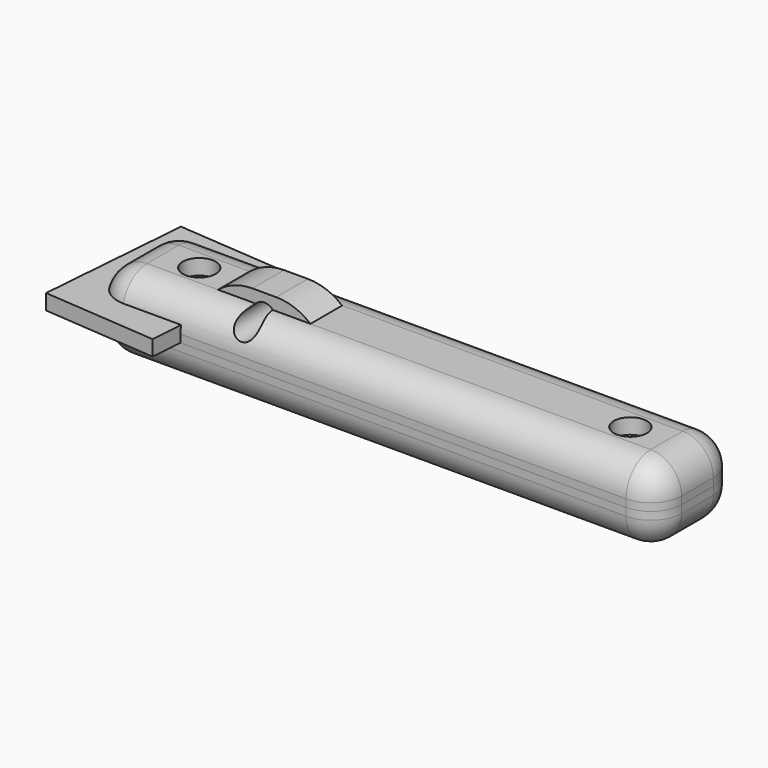
from build123d import *

# Parameters (mm, degrees)
F1_DEPTH    = 2.54
F2_R        = 1.905
F3_DEPTH    = 6.35
F4_DEPTH    = 6.35
F5_R        = 5.08
F6_R        = 5.08
F7_W        = 15.24
F7_H        = 6.5325613847
F8_DEPTH    = 2.032
F9_T1_DEPTH = 34.8168043479
F11_D       = 3.81
F11_DEPTH   = 5.0913193076
F12_D       = 3.81
F14_D       = 5.461
F14_DEPTH   = 2.54
F14_TIP     = 1.6406499203
F15_R       = 1.905
F16_DEPTH   = 4.064


# Not quite as in the source:
# - a fillet or chamfer that OpenCascade refuses, or shapes differently, is made with other operations: its cross-section is extruded or revolved along the edge and cut away or added
# - a feature of the source that left no trace in its solid (it failed there, or was rolled back) is left out


with BuildPart() as f1:
    # F0 (on Top) → F1 (new body)
    with BuildSketch(Plane.XY):
        Polygon((-30.4073522295, 11.7323991549), (-49.1452058091, 13.2097140262), (-50.143391533, 0.5490021481), (-51.1415772568, -12.11170973), (-32.4037236772, -13.5890246013), (-31.6451025271, -3.9668835739), (6.3370331073, -6.9614407455), (6.8161622547, -0.884299044), (-31.1659733796, 2.1102581276), align=None)
        with BuildLine():
            ThreePointArc((-40.386, 0), (-43.2898854466, -2.7918383171), (-45.9653566132, 0.2196008592))
            ThreePointArc((-45.9653566132, 0.2196008592), (-43.0701145534, 2.7918383171), (-40.386, 0))
        make_face(mode=Mode.SUBTRACT)
    extrude(amount=F1_DEPTH)


with BuildPart() as f3:
    # F2 (on Top) → F3 (new body)
    with BuildSketch(Plane.XY):
        Polygon((-46.6201489315, 8.3566), (-46.6201489315, 0), (-46.6201489315, -8.3566), (0, -8.3566), (46.6201489315, -8.3566), (46.6201489315, 0), (46.6201489315, 8.3566), (0, 8.3566), align=None)
        with BuildLine():
            ThreePointArc((-37.465, 0), (-35.56, 1.905), (-33.655, 0))
            ThreePointArc((-33.655, 0), (-35.56, -1.905), (-37.465, 0))
        make_face(mode=Mode.SUBTRACT)
        with Locations((35.56, 0)):
            Circle(F2_R, mode=Mode.SUBTRACT)
    extrude(amount=F3_DEPTH)

    # F5
    f5_edges = [f3.edges().sort_by_distance(p)[0] for p in [
        (0, -8.3566, 6.35),
        (-46.620149, 0, 6.35),
        (0, 8.3566, 6.35),
        (46.620149, 0, 6.35),
        (-46.620149, -8.3566, 3.175),
        (-46.620149, 8.3566, 3.175),
        (46.620149, -8.3566, 3.175),
        (46.620149, 8.3566, 3.175),
    ]]
    fillet(f5_edges, radius=F5_R)

    # F7 (on face) → F8 (join)
    with BuildSketch(Plane.XY.offset(6.35)):
        with Locations((-22.225, 0)):
            Rectangle(F7_W, F7_H)
    extrude(amount=F8_DEPTH)

    # F9: fillet of radius 8.89 on 2 edges, made by hand

    # F9_s2 → F9_t1 (cut)
    with BuildSketch(Plane.XZ.offset(-17.408402174)):
        with BuildLine():
            ThreePointArc((-29.845, 6.35), (-27.1935199372, 7.8585918987), (-24.1881514074, 8.382))
            Line((-24.1881514074, 8.382), (-29.845, 8.382))
            Line((-29.845, 8.382), (-29.845, 6.35))
        make_face()
        with BuildLine():
            ThreePointArc((-14.605, 6.35), (-17.2564800628, 7.8585918987), (-20.2618485926, 8.382))
            Line((-20.2618485926, 8.382), (-14.605, 8.382))
            Line((-14.605, 8.382), (-14.605, 6.35))
        make_face()
    extrude(amount=F9_T1_DEPTH, mode=Mode.SUBTRACT)

    # F11 (through all, one way)
    with BuildSketch(Plane(origin=(0, -3.2662806924, 0), x_dir=(1, 0, 0), z_dir=(0, 1, 0))):
        with Locations((-22.225, -5.08)):
            Circle(F11_D / 2)
    extrude(amount=-F11_DEPTH, mode=Mode.SUBTRACT)

    # F12 (through all)
    with Locations(Plane.XZ.offset(3.2662806924)):
        with Locations((-22.225, 5.08)):
            Hole(F12_D / 2)

    # F14
    with Locations(Plane.XY.offset(6.35)):
        with Locations((35.56, 0), (-35.56, 0)):
            Hole(F14_D / 2, depth=F14_DEPTH)
            with Locations((0, 0, -(F14_DEPTH + F14_TIP / 2))):  # 118° drill point
                Cone(0, F14_D / 2, F14_TIP, mode=Mode.SUBTRACT)


with BuildPart() as f4:
    # F2 (on Top) → F4 (new body)
    with BuildSketch(Plane.XY):
        Polygon((-46.6201489315, 8.3566), (-46.6201489315, 0), (-46.6201489315, -8.3566), (0, -8.3566), (46.6201489315, -8.3566), (46.6201489315, 0), (46.6201489315, 8.3566), (0, 8.3566), align=None)
        with BuildLine():
            ThreePointArc((-37.465, 0), (-35.56, 1.905), (-33.655, 0))
            ThreePointArc((-33.655, 0), (-35.56, -1.905), (-37.465, 0))
        make_face(mode=Mode.SUBTRACT)
        with Locations((35.56, 0)):
            Circle(F2_R, mode=Mode.SUBTRACT)
    extrude(amount=-F4_DEPTH)

    # F6
    f6_edges = [f4.edges().sort_by_distance(p)[0] for p in [
        (-46.620149, 0, -6.35),
        (0, -8.3566, -6.35),
        (46.620149, 0, -6.35),
        (0, 8.3566, -6.35),
        (46.620149, -8.3566, -3.175),
        (46.620149, 8.3566, -3.175),
        (-46.620149, -8.3566, -3.175),
        (-46.620149, 8.3566, -3.175),
    ]]
    fillet(f6_edges, radius=F6_R)

    # F15 (on face) → F16 (cut)
    with BuildSketch(Plane(origin=(0, 0, -6.35), x_dir=(1, 0, 0), z_dir=(0, 0, -1))):
        Polygon((-33.98354509, -2.7305), (-32.40709018, 0), (-33.98354509, 2.7305), (-37.13645491, 2.7305), (-38.71290982, 0), (-37.13645491, -2.7305), align=None)
        with Locations((-35.56, 0)):
            Circle(F15_R, mode=Mode.SUBTRACT)
        Polygon((37.13645491, -2.7305), (38.71290982, 0), (37.13645491, 2.7305), (33.98354509, 2.7305), (32.40709018, 0), (33.98354509, -2.7305), align=None)
        with Locations((35.56, 0)):
            Circle(F15_R, mode=Mode.SUBTRACT)
    extrude(amount=-F16_DEPTH, mode=Mode.SUBTRACT)


solid = Compound([f1.part, f3.part, f4.part])
